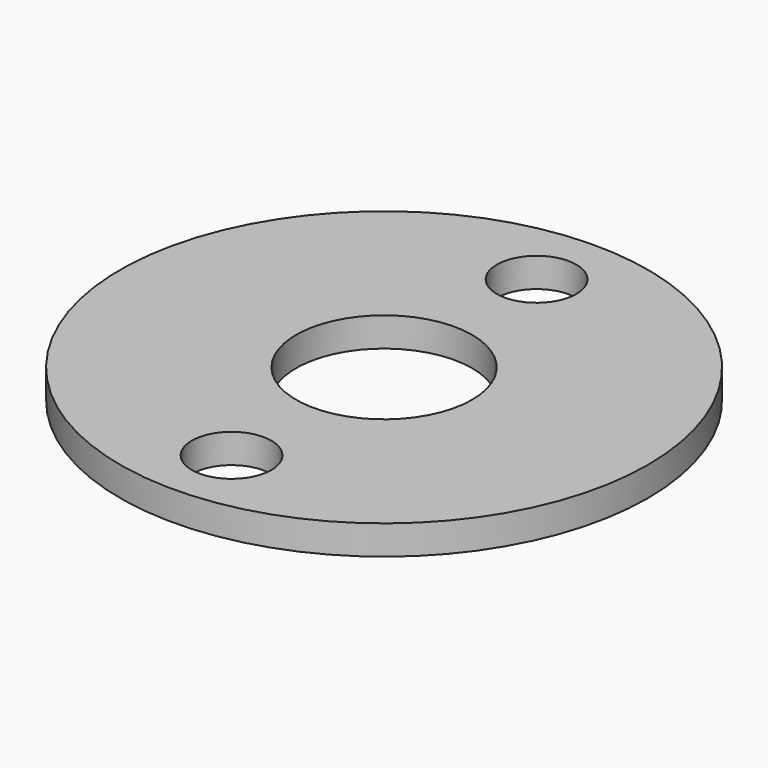
from build123d import *

# Parameters (mm, degrees)
F0_R     = 14.2875
F0_R_2   = 2.15265
F0_R_3   = 4.7625
F1_DEPTH = 1.5875


# Not quite as in the source:
# - a feature names something its author has since deleted; it is built from what else it names


with BuildPart() as f1:
    # F0 (on Top) → F1 (new body)
    with BuildSketch(Plane.XY):
        Circle(F0_R)
        with Locations((0, -10.31875)):
            Circle(F0_R_2, mode=Mode.SUBTRACT)
        Circle(F0_R_3, mode=Mode.SUBTRACT)
        with Locations((0, 10.31875)):
            Circle(F0_R_2, mode=Mode.SUBTRACT)
    extrude(amount=F1_DEPTH)


solid = f1.part
